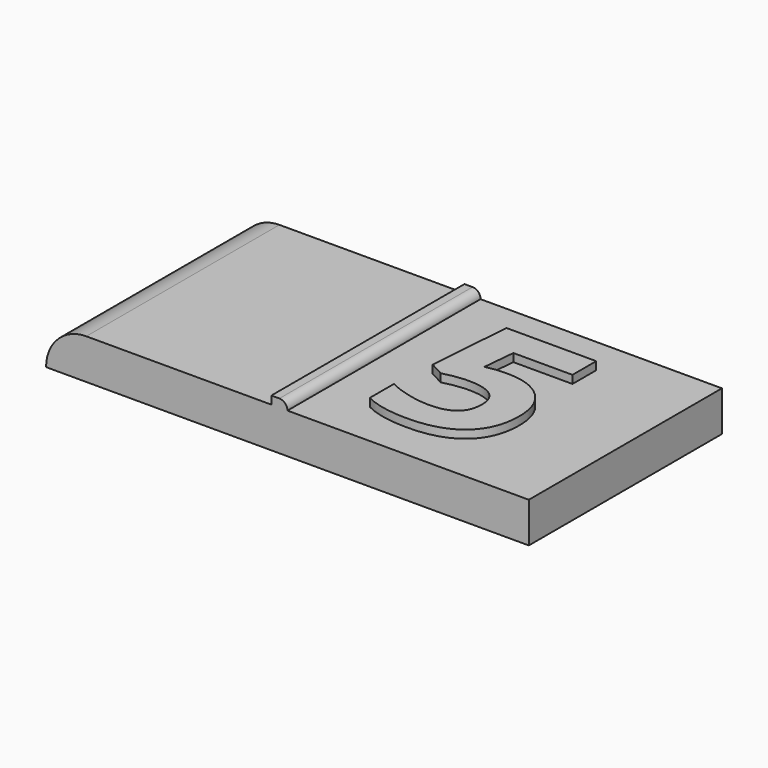
from build123d import *

# Parameters (mm, degrees)
F0_W         = 60
F0_H         = 30
F1_DEPTH     = 5
F2_W         = 2
F2_H         = 30
F3_DEPTH     = 1
F4_R         = 0.99999
F5_TEXT_SIZE = 28.8201948731
F6_DEPTH     = 1
F7_R         = 4.99999


# Not quite as in the source:
# - a fillet or chamfer is up to 0.001 mm smaller than in the source, because OpenCascade refuses the exact size
# - Text() gives the source's letters only with a copy of the font that has no kerning and outlines rounded to 1/6400 em; it was checked with that copy


with BuildPart() as f1:
    # F0 (on Top) → F1 (new body)
    with BuildSketch(Plane.XY):
        with Locations((30, 15)):
            Rectangle(F0_W, F0_H)
    extrude(amount=F1_DEPTH)

    # F2 (on face) → F3 (join)
    with BuildSketch(Plane.XY.offset(5)):
        with Locations((29, 15)):
            Rectangle(F2_W, F2_H)
    extrude(amount=F3_DEPTH)

    # F4 (radius 1 in the source; OpenCascade refuses exactly that, so slightly less here)
    f4_edges = [f1.edges().sort_by_distance(p)[0] for p in [
        (30, 15, 6),
    ]]
    fillet(f4_edges, radius=F4_R)

    # F5 (on face) → F6 (join)
    with BuildSketch(Plane.XY.offset(5)):
        with Locations((34.3574509025, 4.7624194995)):
            Text('5', F5_TEXT_SIZE, font='Open Sans', font_style=FontStyle.BOLD, text_align=(TextAlign.LEFT, TextAlign.BOTTOM))
    extrude(amount=F6_DEPTH)

    # F7 (radius 5 in the source; OpenCascade refuses exactly that, so slightly less here)
    f7_edges = [f1.edges().sort_by_distance(p)[0] for p in [
        (0, 15, 5),
    ]]
    fillet(f7_edges, radius=F7_R)


solid = f1.part
